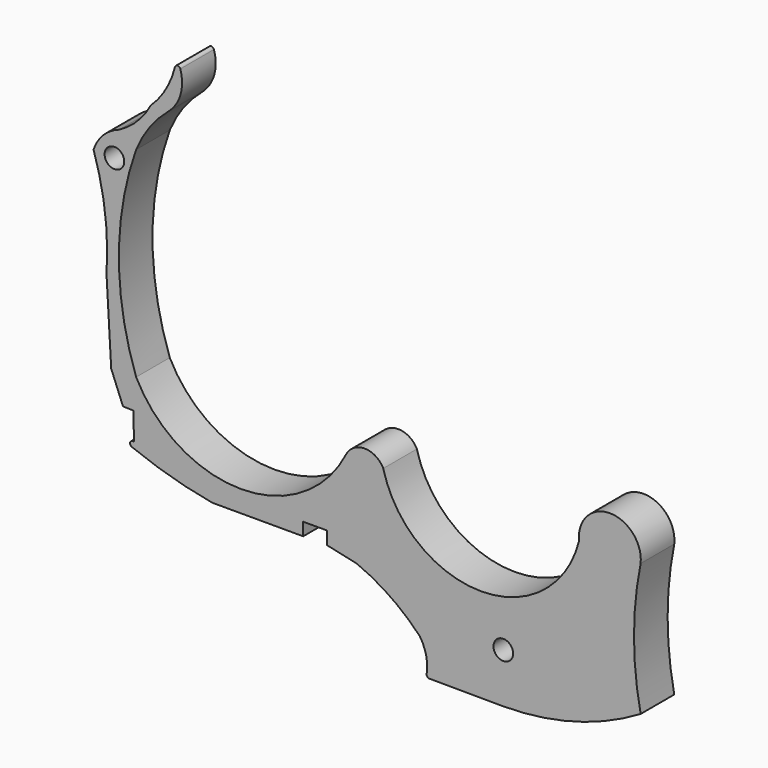
from build123d import *

# Parameters (mm, degrees)
F1_DEPTH = 3.81
F2_R     = 0.254
F3_D     = 1.778


# Not quite as in the source:
# - a feature names something its author has since deleted; it is built from what else it names


with BuildPart() as f1:
    # F0 (on Front) → F1 (new body)
    with BuildSketch(Plane.XZ):
        with BuildLine():
            ThreePointArc((41.4086468518, -4.477661373), (40.8064485211, 1.5249027452), (41.4086468518, 7.5274668634))
            ThreePointArc((41.4086468518, 7.5274668634), (38.62243375, 10.6323405578), (35.8362206482, 7.5274668634))
            ThreePointArc((35.8362206482, 7.5274668634), (26.9629642945, 0.6052852493), (18.0897079408, 7.5274668634))
            ThreePointArc((18.0897079408, 7.5274668634), (16.3997087002, 8.5658356165), (14.7097094595, 7.5274668634))
            ThreePointArc((14.7097094595, 7.5274668634), (5.20431123, 1.6871633473), (-4.3010869995, 7.5274668634))
            ThreePointArc((-4.3010869995, 7.5274668634), (-5.8660457098, 16.6021063924), (-4.3010869995, 25.6767459214))
            ThreePointArc((-4.3010869995, 25.6767459214), (-3.0718420066, 27.8672574596), (-1.3499599881, 29.6960566193))
            ThreePointArc((-1.3499599881, 29.6960566193), (-0.1811880249, 31.805372823), (-0.6376186502, 34.1732650995))
            ThreePointArc((-0.6376186502, 34.1732650995), (-1.421034245, 31.7066061173), (-2.9725597706, 29.6351537108))
            ThreePointArc((-2.9725597706, 29.6351537108), (-4.1943946694, 27.9789305778), (-5.8506173082, 26.7570950091))
            ThreePointArc((-5.8506173082, 26.7570950091), (-7.277149178, 25.8612568479), (-8.1605734304, 24.4270041585))
            ThreePointArc((-8.1605734304, 24.4270041585), (-7.1141917577, 19.7155957013), (-6.9871647283, 14.8910596211))
            Line((-6.9871647283, 14.8910596211), (-6.5609117303, 7.4617798516))
            Line((-6.5609117303, 7.4617798516), (-5.4928543977, 4.8075970262))
            Line((-5.4928543977, 4.8075970262), (-4.555047024, 4.7773430124))
            Line((-4.555047024, 4.7773430124), (-4.4945431873, 2.3267425131))
            Line((-4.4945431873, 2.3267425131), (-5.734869279, 2.2662337869))
            ThreePointArc((-5.734869279, 2.2662337869), (-1.646496666, 0.760301383), (2.5915002188, -0.2506414603))
            Line((2.5915002188, -0.2506414603), (10.8333304524, -0.2506414603))
            Line((10.8333304524, -0.2506414603), (10.8333304524, 0.9162292117))
            Line((10.8333304524, 0.9162292117), (12.9701783881, 0.9162292117))
            Line((12.9701783881, 0.9162292117), (12.9701783881, -0.2506414603))
            Line((12.9701783881, -0.2506414603), (15.6823657453, -0.8442893741))
            ThreePointArc((15.6823657453, -0.8442893741), (18.751499307, -2.5127162084), (21.4028581977, -4.7872546129))
            ThreePointArc((21.4028581977, -4.7872546129), (22.004430538, -6.2762052491), (21.9660382718, -7.8816302121))
            Line((21.9660382718, -7.8816302121), (28.9244800806, -7.9146586359))
            ThreePointArc((28.9244800806, -7.9146586359), (35.3988018628, -7.0397169385), (41.4086468518, -4.477661373))
        make_face()
    extrude(amount=F1_DEPTH)

    # F2
    f2_edges = [f1.edges().sort_by_distance(p)[0] for p in [
        (-0.637619, -1.905, 34.173265),
        (21.966038, -1.905, -7.88163),
        (-5.734869, -1.905, 2.266234),
    ]]
    fillet(f2_edges, radius=F2_R)

    # F3 (through all)
    with Locations(Plane(origin=(0, 0, 0), x_dir=(1, 0, 0), z_dir=(0, 1, 0))):
        with Locations((28.9652328938, 3.4148474224), (-6.2686339952, -24.3659485132)):
            Hole(F3_D / 2)


solid = f1.part
